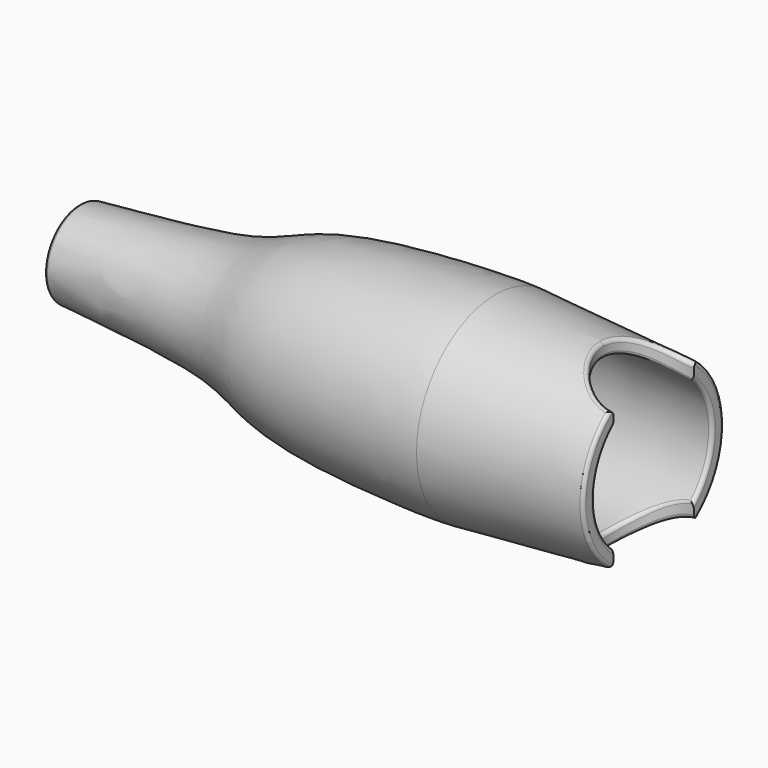
from build123d import *

# Parameters (mm, degrees)
F3_DEPTH = 15
F4_R     = 0.5


with BuildPart() as f1:
    # F0 (on Front) → F1 (revolve)
    with BuildSketch(Plane.XZ):
        with BuildLine():
            Line((80, 12.2116101372), (58, 13.75))
            add(Edge.make_bspline(
                [(0, 6), (11.5316812488, 6.9890408187), (23.1095059085, 7.654299135), (32.4265124844, 13.2991909742), (54.4413961611, 13.9988418214), (58, 13.75)],
                knots=[0, 0, 0, 0, 0.368705424, 0.6258372181, 1, 1, 1, 1], degree=3))
            Line((0, 6), (0, 5))
            add(Edge.make_bspline(
                [(0, 5), (16.5526148169, 5.9873342484), (25.2846415733, 7.250504946), (33.4289631457, 10.9050283003), (54.4214783481, 12.1981144433), (58, 11.75)],
                knots=[0, 0, 0, 0, 0.3973878043, 0.6244343912, 1, 1, 1, 1], degree=3))
            Line((58, 11.75), (80, 10.2116101372))
            Line((80, 10.2116101372), (80, 12.2116101372))
        make_face()
    revolve(axis=Axis((24.9500407372, 0, 0), (1, 0, 0)))

    # F2 (on Top) → F3 (cut, symmetric)
    with BuildSketch(Plane.XY):
        with BuildLine():
            Line((80, -7), (80, 7))
            ThreePointArc((80, 7), (73, 0), (80, -7))
        make_face()
    extrude(amount=F3_DEPTH, both=True, mode=Mode.SUBTRACT)

    # F4
    f4_edges = [f1.edges().sort_by_distance(p)[0] for p in [
        (75.076094, -4.975455, 11.528055),
        (75.076094, 4.975455, 11.528055),
        (73, 0, -12.701098),
        (75.092909, -4.992039, 9.299583),
        (73, 0, -10.701098),
        (75.092909, 4.992039, 9.299583),
        (80, 12.21161, 0),
        (80, -12.21161, 0),
        (80, 10.21161, 0),
        (80, -10.21161, 0),
        (0, 0, -6),
        (0, 0, -5),
    ]]
    fillet(f4_edges, radius=F4_R)


solid = f1.part
